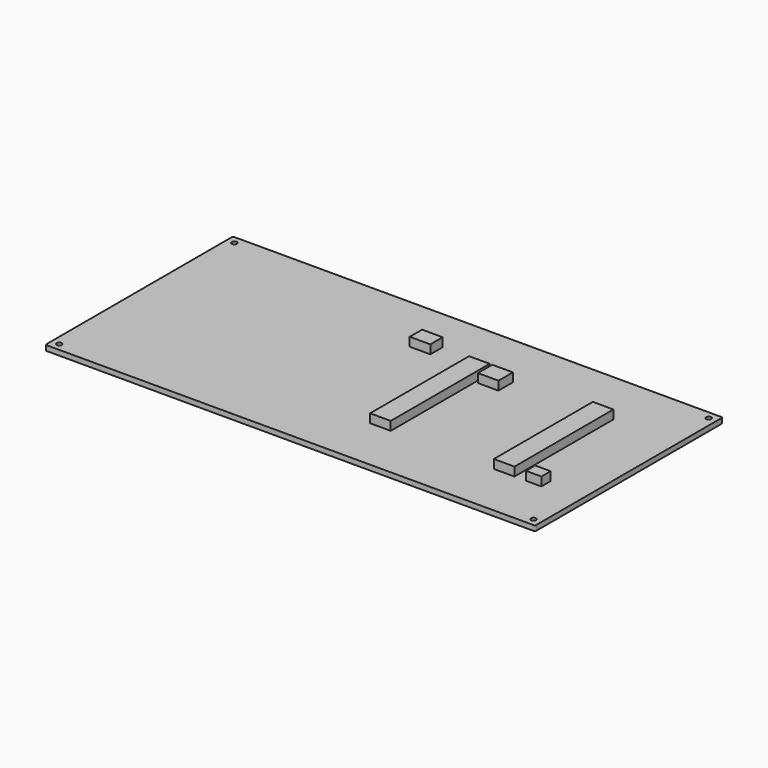
from build123d import *

# Parameters (mm, degrees)
F0_W      = 190
F0_H      = 90.933
F1_DEPTH  = 2
F2_R      = 1
F3_DEPTH  = 2.001
F6_R      = 0.5
F7_W      = 8
F7_H      = 48
F7_H_2    = 7
F8_DEPTH  = 3.4
F9_W      = 8
F9_H      = 6
F10_DEPTH = 3.4


# Not quite as in the source:
# - a feature names something its author has since deleted; it is built from what else it names


with BuildPart() as f1:
    # F0 (on Top) → F1 (new body)
    with BuildSketch(Plane.XY):
        with Locations((95, 45.4665)):
            Rectangle(F0_W, F0_H)
    extrude(amount=F1_DEPTH)

    # F2 (on face) → F3 (cut, through all)
    with BuildSketch(Plane.XY.offset(2)):
        with Locations((3, 87.933)):
            Circle(F2_R)
        with Locations((3, 3)):
            Circle(F2_R)
    f3 = extrude(amount=-F3_DEPTH, mode=Mode.SUBTRACT)

    # F5: F3 across plane
    add(f3.mirror(Plane(origin=(95, 45.4665, 1), x_dir=(0, -1, 0), z_dir=(-1, 0, 0))), mode=Mode.SUBTRACT)

    # F6
    f6_edges = [f1.edges().sort_by_distance(p)[0] for p in [
        (190, 0, 1),
        (190, 90.933, 1),
        (0, 90.933, 1),
        (0, 0, 1),
    ]]
    fillet(f6_edges, radius=F6_R)

    # F7 (on face) → F8 (join)
    with BuildSketch(Plane.XY.offset(2)):
        with Locations((113, 45.233)):
            Rectangle(F7_W, F7_H)
        with Locations((161, 45.233)):
            Rectangle(F7_W, F7_H)
        with Locations((122, 65.733)):
            Rectangle(F7_W, F7_H_2)
        Polygon((169.4320317507, 25.7526094498), (169.4320317507, 21.2526094498), (175.4320317507, 21.2526094498), (175.4320317507, 25.6957146213), align=None)
    extrude(amount=F8_DEPTH)

    # F9 (on face) → F10 (join)
    with BuildSketch(Plane.XY.offset(2)):
        with Locations((91, 70.933)):
            Rectangle(F9_W, F9_H)
    extrude(amount=F10_DEPTH)


solid = f1.part
